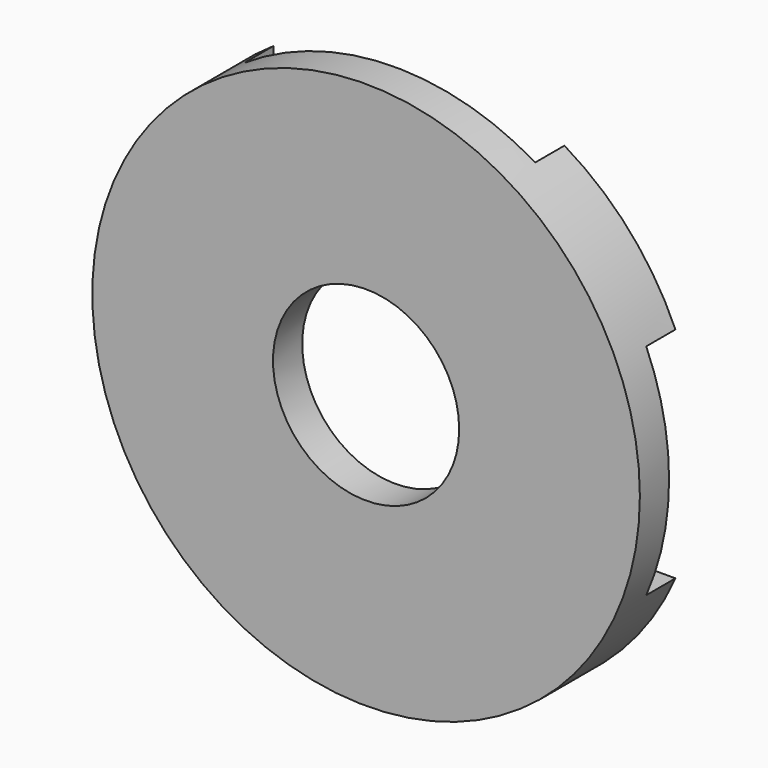
from build123d import *

# Parameters (mm, degrees)
F0_R          = 12.7
F1_DEPTH      = 17.78
F2_R          = 38.1
F3_DEPTH      = 10.16
F4_R          = 12.954
F5_DEPTH      = 17.781
F5_DEPTH_BACK = 115
F6_W          = 5.08
F6_H          = 30.48
F7_DEPTH      = 38.101
F7_DEPTH_BACK = 38.101
F8_W          = 40.513
F8_H          = 5.08
F9_DEPTH      = 38.101
F9_DEPTH_BACK = 38.101


# Not quite as in the source:
# - an extrude ends at something that could not be found from the text; its depth is read off the source's solid


with BuildPart() as f1:
    # F0 (on Front) → F1 (new body)
    with BuildSketch(Plane.XZ):
        Circle(F0_R)
    extrude(amount=F1_DEPTH)

    # F2 (on Front) → F3 (join)
    with BuildSketch(Plane.XZ):
        Circle(F2_R)
    extrude(amount=F3_DEPTH)

    # F4 (on Front) → F5 (cut, two sides)
    with BuildSketch(Plane.XZ) as f5_sk:
        Circle(F4_R)
    extrude(amount=F5_DEPTH, mode=Mode.SUBTRACT)
    extrude(f5_sk.sketch, amount=-F5_DEPTH_BACK, mode=Mode.SUBTRACT)

    # F6 (on Right) → F7 (cut, two sides)
    with BuildSketch(Plane.YZ) as f7_sk:
        with Locations((-2.54, 0)):
            Rectangle(F6_W, F6_H)
    extrude(amount=F7_DEPTH, mode=Mode.SUBTRACT)
    extrude(f7_sk.sketch, amount=-F7_DEPTH_BACK, mode=Mode.SUBTRACT)

    # F8 (on Top) → F9 (cut, two sides)
    with BuildSketch(Plane.XY) as f9_sk:
        with Locations((-0.7823046945, -2.54)):
            Rectangle(F8_W, F8_H)
    extrude(amount=-F9_DEPTH, mode=Mode.SUBTRACT)
    extrude(f9_sk.sketch, amount=F9_DEPTH_BACK, mode=Mode.SUBTRACT)


solid = f1.part
